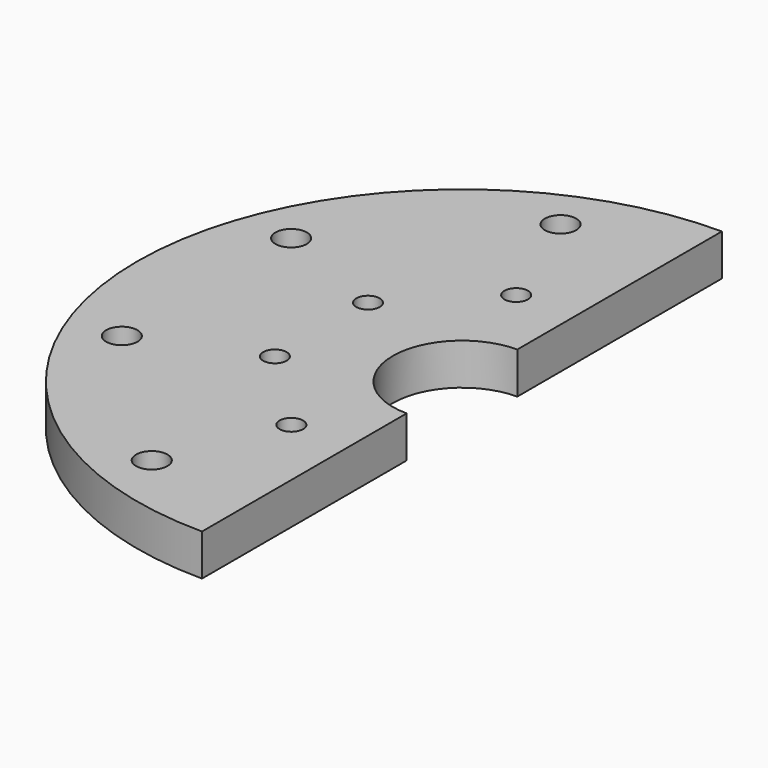
from build123d import *

# Parameters (mm, degrees)
F0_R     = 74.6125
F1_DEPTH = 9.525
F2_R     = 15.875
F3_DEPTH = 9.526
F5_D     = 5.4
F6_R     = 2.7
F7_DEPTH = 9.526
F9_D     = 7.2


with BuildPart() as f1:
    # F0 (on Top) → F1 (new body)
    with BuildSketch(Plane.XY):
        Circle(F0_R)
    extrude(amount=F1_DEPTH)

    # F2 (on face) → F3 (cut, through all)
    with BuildSketch(Plane.XY.offset(9.525)):
        Circle(F2_R)
    extrude(amount=-F3_DEPTH, mode=Mode.SUBTRACT)

    # F5 (through all)
    with Locations(Plane.XY.offset(9.525)):
        with Locations((-13.3652133, 32.2664949823), (-32.2664903636, 13.3652244507), (-32.2664949823, -13.3652133), (-13.3652244507, -32.2664903636), (13.3652133, -32.2664949823), (32.2664903636, -13.3652244507), (32.2664949823, 13.3652133), (13.3652244507, 32.2664903636)):
            Hole(F5_D / 2)

    # F6 (on face) → F7 (cut, through all)
    with BuildSketch(Plane.XY.offset(9.525)):
        with BuildLine():
            Line((92.0014753938, 88.4870588779), (0, 88.4870588779))
            Line((0, 88.4870588779), (0, 74.6125))
            ThreePointArc((0, 74.6125), (52.7590047113, 52.7590047113), (74.6125, 0))
            ThreePointArc((74.6125, 0), (52.7590047113, -52.7590047113), (0, -74.6125))
            Line((0, -74.6125), (0, -93.3939293027))
            Line((0, -93.3939293027), (92.0014753938, -93.3939293027))
            Line((92.0014753938, -93.3939293027), (92.0014753938, 88.4870588779))
        make_face()
        with BuildLine():
            ThreePointArc((74.6125, 0), (52.7590047113, 52.7590047113), (0, 74.6125))
            Line((0, 74.6125), (0, 15.875))
            ThreePointArc((0, 15.875), (11.2253201513, 11.2253201513), (15.875, 0))
            ThreePointArc((15.875, 0), (11.2253201513, -11.2253201513), (0, -15.875))
            Line((0, -15.875), (0, -74.6125))
            ThreePointArc((0, -74.6125), (52.7590047113, -52.7590047113), (74.6125, 0))
        make_face()
        with Locations((13.3652133, -32.2664949823)):
            Circle(F6_R, mode=Mode.SUBTRACT)
        with Locations((32.2664903636, -13.3652244507)):
            Circle(F6_R, mode=Mode.SUBTRACT)
        with Locations((32.2664949823, 13.3652133)):
            Circle(F6_R, mode=Mode.SUBTRACT)
        with Locations((13.3652244507, 32.2664903636)):
            Circle(F6_R, mode=Mode.SUBTRACT)
    extrude(amount=-F7_DEPTH, mode=Mode.SUBTRACT)

    # F9 (through all)
    with Locations(Plane.XY.offset(9.525)):
        with Locations((-24.300392725, 58.6663524809), (-58.6663481481, 24.3004031854), (-58.6663524809, -24.300392725), (-24.3004031854, -58.6663481481)):
            Hole(F9_D / 2)


solid = f1.part
